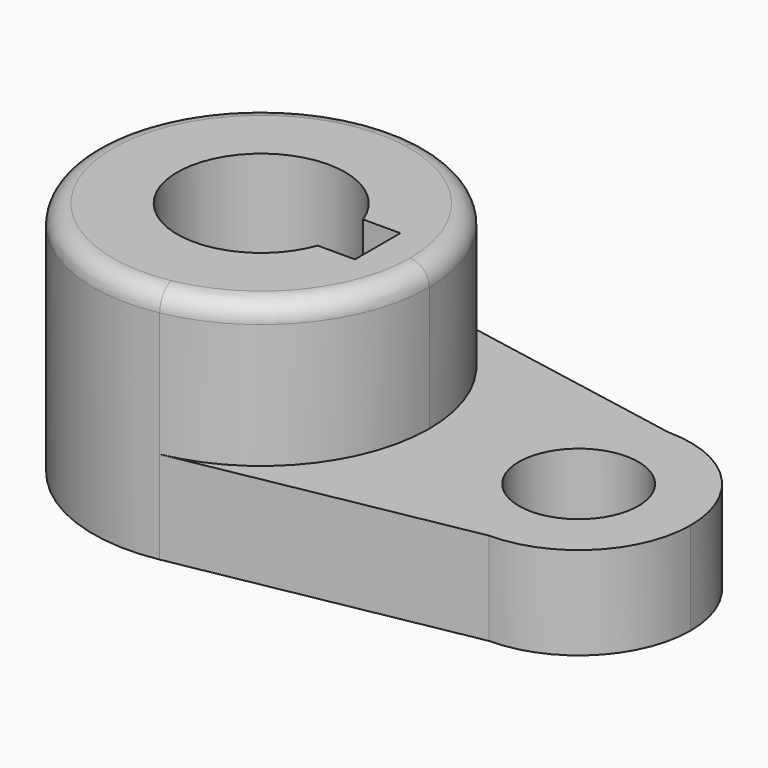
from build123d import *

# Parameters (mm, degrees)
F1_DEPTH = 40.2336
F2_DEPTH = 15.7734
F3_R     = 3.302


# Not quite as in the source:
# - a feature names something its author has since deleted; it is built from what else it names


with BuildPart() as f1:
    # F0 (on Top) → F1 (new body)
    with BuildSketch(Plane.XY):
        with BuildLine():
            ThreePointArc((5.2118165727, -28.0956863773), (21.9710978739, -18.2702348977), (28.575, 0))
            ThreePointArc((28.575, 0), (21.9710978739, 18.2702348977), (5.2118165727, 28.0956863773))
            ThreePointArc((5.2118165727, 28.0956863773), (-28.575, 0), (5.2118165727, -28.0956863773))
        make_face()
        with BuildLine():
            ThreePointArc((13.4477648793, -4.826), (-14.2875, 0), (13.4477648793, 4.826))
            Line((13.4477648793, 4.826), (19.7977648793, 4.826))
            Line((19.7977648793, 4.826), (19.7977648793, 0))
            Line((19.7977648793, 0), (19.7977648793, -4.826))
            Line((19.7977648793, -4.826), (13.4477648793, -4.826))
        make_face(mode=Mode.SUBTRACT)
    extrude(amount=F1_DEPTH)

    # F0 (on Top) → F2 (join)
    with BuildSketch(Plane.XY):
        with BuildLine():
            ThreePointArc((5.2118165727, 28.0956863773), (21.9710978739, 18.2702348977), (28.575, 0))
            Line((28.575, 0), (34.925, 0))
            ThreePointArc((34.925, 0), (40.5046158184, 13.4703841816), (53.975, 19.05))
            Line((53.975, 19.05), (5.2118165727, 28.0956863773))
        make_face()
        with BuildLine():
            Line((34.925, 0), (28.575, 0))
            ThreePointArc((28.575, 0), (21.9710978739, -18.2702348977), (5.2118165727, -28.0956863773))
            Line((5.2118165727, -28.0956863773), (53.975, -19.05))
            ThreePointArc((53.975, -19.05), (40.5046158184, -13.4703841816), (34.925, 0))
        make_face()
        with BuildLine():
            ThreePointArc((53.975, 19.05), (40.5046158184, 13.4703841816), (34.925, 0))
            ThreePointArc((34.925, 0), (40.5046158184, -13.4703841816), (53.975, -19.05))
            ThreePointArc((53.975, -19.05), (67.4453841816, -13.4703841816), (73.025, 0))
            ThreePointArc((73.025, 0), (67.4453841816, 13.4703841816), (53.975, 19.05))
        make_face()
        with BuildLine():
            ThreePointArc((64.135, 0), (53.975, -10.16), (43.815, 0))
            ThreePointArc((43.815, 0), (53.975, 10.16), (64.135, 0))
        make_face(mode=Mode.SUBTRACT)
    extrude(amount=F2_DEPTH)

    # F3
    f3_edges = [f1.edges().sort_by_distance(p)[0] for p in [
        (-5.211817, 28.095686, 40.2336),
    ]]
    fillet(f3_edges, radius=F3_R)


solid = f1.part
